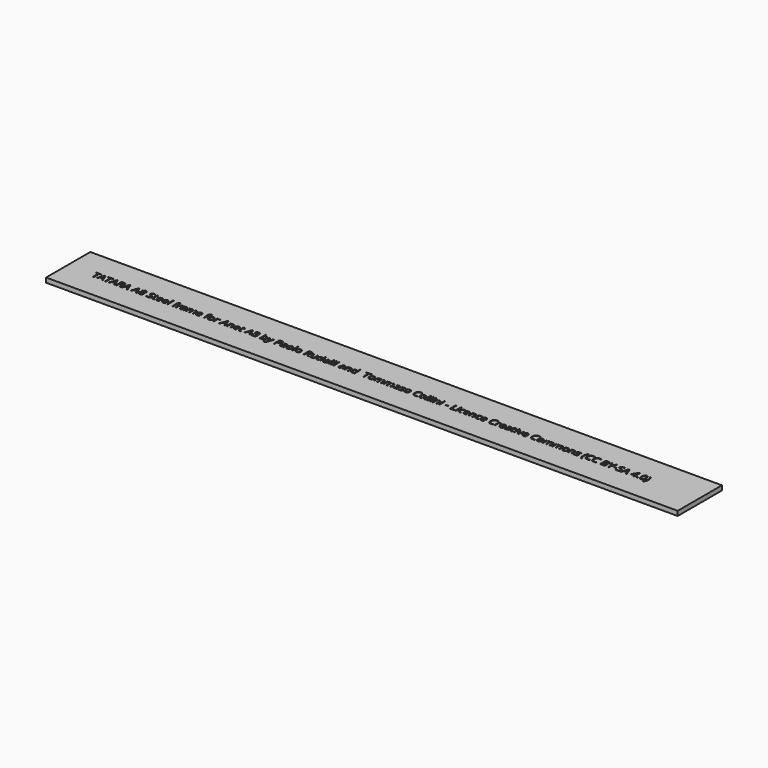
from build123d import *

# Parameters (mm, degrees)
F0_TEXT_SIZE = 26.7251161858
F2_DEPTH     = 25
F3_START     = 6
F1_W         = 1650
F1_H         = 144.4578327995
F3_DEPTH     = 12


# Not quite as in the source:
# - Text() gives the source's letters only with a copy of the font that has no kerning and outlines rounded to 1/6400 em; it was checked with that copy


with BuildPart() as f2:
    # F0 (on Top) → F2 (new body)
    with BuildSketch(Plane.XY):
        with Locations((-564.9470686913, -10.9999980778)):
            Text('TATARA A8 Steel frame for Anet A8 by Paolo Rudelli and  Tommaso Collini - Licence Creative Commons (CC BY-SA 4.0)', F0_TEXT_SIZE, font='Open Sans', text_align=(TextAlign.LEFT, TextAlign.BOTTOM))
    extrude(amount=F2_DEPTH)


with BuildPart() as f3:
    # F1 (on Top) → F3 (new body)
    with BuildSketch(Plane.XY.offset(F3_START)):
        with Locations((193.6645805836, -0.9821914136)):
            Rectangle(F1_W, F1_H)
    extrude(amount=F3_DEPTH)

    # F4: cut F2
    add(f2.part, mode=Mode.SUBTRACT)


solid = f3.part
